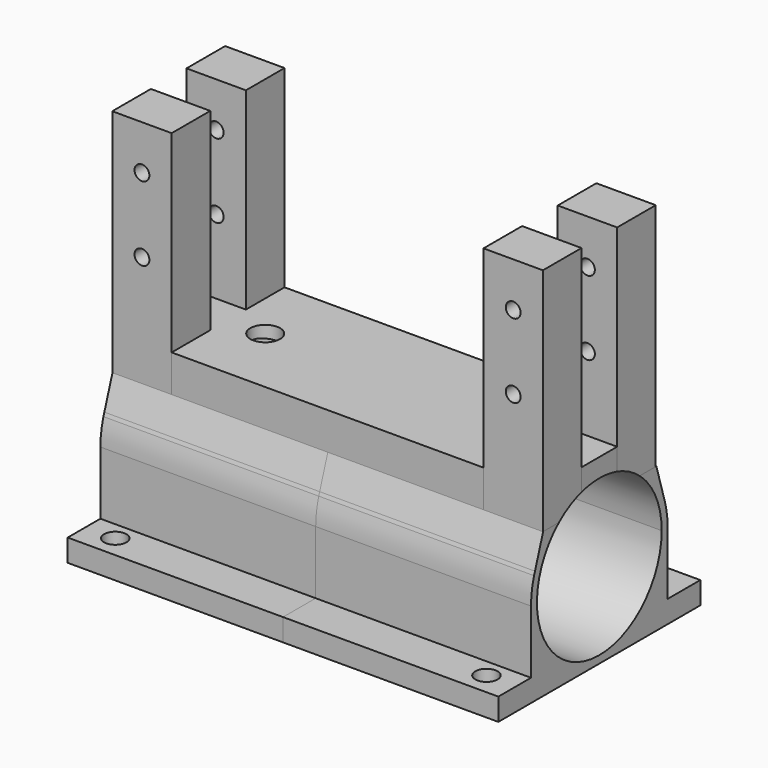
from build123d import *

# Parameters (mm, degrees)
F0_W      = 8
F0_H      = 6.5
F1_DEPTH  = 31
F0_R      = 2
F2_DEPTH  = 5
F3_R      = 1
F4_DEPTH  = 12.5
F5_W      = 5.5
F5_H      = 3
F6_DEPTH  = 29
F9_R      = 10.5
F10_DEPTH = 83.001
F0_R_2    = 1.5
F11_DEPTH = 19.501


# Not quite as in the source:
# - the program builds the solid bodies; features that only make, move or delete a surface that nothing else refers to are left out


with BuildPart() as f1:
    # F0 (on Top) → F1 (new body)
    with BuildSketch(Plane.XY):
        with Locations((-25, 6.25)):
            Rectangle(F0_W, F0_H)
    extrude(amount=F1_DEPTH)


with BuildPart() as f1b:
    # F0 (on Top) → F1, piece 2 (new body)
    with BuildSketch(Plane.XY):
        with Locations((-25, -6.25)):
            Rectangle(F0_W, F0_H)
    extrude(amount=F1_DEPTH)


with BuildPart() as f1c:
    # F0 (on Top) → F1, piece 3 (new body)
    with BuildSketch(Plane.XY):
        with Locations((25, 6.25)):
            Rectangle(F0_W, F0_H)
    extrude(amount=F1_DEPTH)


with BuildPart() as f1d:
    # F0 (on Top) → F1, piece 4 (new body)
    with BuildSketch(Plane.XY):
        with Locations((25, -6.25)):
            Rectangle(F0_W, F0_H)
    extrude(amount=F1_DEPTH)


with BuildPart() as f2:
    # F0 (on Top) → F2 (new body)
    with BuildSketch(Plane.XY):
        Polygon((-21, -9.5), (21, -9.5), (21, -3), (29, -3), (29, 3), (21, 3), (21, 9.5), (-21, 9.5), (-21, 3), (-29, 3), (-29, -3), (-21, -3), align=None)
        with Locations((-16, 0)):
            Circle(F0_R, mode=Mode.SUBTRACT)
        with Locations((16, 0)):
            Circle(F0_R, mode=Mode.SUBTRACT)
    extrude(amount=F2_DEPTH)


with BuildPart() as f4_tool:
    # F3 (on Front) → F4 (new body, symmetric)
    with BuildSketch(Plane.XZ):
        with Locations((25, 25)):
            Circle(F3_R)
        with Locations((25, 15)):
            Circle(F3_R)
        with Locations((-25, 25)):
            Circle(F3_R)
        with Locations((-25, 15)):
            Circle(F3_R)
    extrude(amount=F4_DEPTH, both=True)


with BuildPart() as f1_1:
    add(f1.part)

    # F4: cut by f4_tool
    add(f4_tool.part, mode=Mode.SUBTRACT)


with BuildPart() as f1b_1:
    add(f1b.part)

    # F4: cut by f4_tool
    add(f4_tool.part, mode=Mode.SUBTRACT)


with BuildPart() as f1c_1:
    add(f1c.part)

    # F4: cut by f4_tool
    add(f4_tool.part, mode=Mode.SUBTRACT)


with BuildPart() as f1d_1:
    add(f1d.part)

    # F4: cut by f4_tool
    add(f4_tool.part, mode=Mode.SUBTRACT)


with BuildPart() as f6:
    # F5 (on Right) → F6 (new body, symmetric)
    with BuildSketch(Plane.YZ):
        with BuildLine():
            ThreePointArc((-10.8310090403, -4.1348682857), (-9.7674911279, -1.9298997482), (-8.2613558209, 0))
            Line((-8.2613558209, 0), (-9.4548137859, 0))
            Line((-9.4548137859, 0), (-10.8310090403, -4.1348682857))
        make_face()
        with BuildLine():
            ThreePointArc((6.8007352544, 0), (9.5304176239, -3.5930577591), (10.5, -8))
            ThreePointArc((10.5, -8), (-4.4069422409, -17.5304176239), (-6.8007352544, 0))
            Line((-6.8007352544, 0), (-8.2613558209, 0))
            ThreePointArc((-8.2613558209, 0), (-9.7674911279, -1.9298997482), (-10.8310090403, -4.1348682857))
            Line((-10.8310090403, -4.1348682857), (-10.9869876699, -4.6035162385))
            ThreePointArc((-10.9869876699, -4.6035162385), (-11.3710236611, -6.2824957356), (-11.5, -8))
            ThreePointArc((-11.5, -8), (-8.1317279836, -16.1317279836), (0, -19.5))
            ThreePointArc((0, -19.5), (8.1317279836, -16.1317279836), (11.5, -8))
            ThreePointArc((11.5, -8), (11.3918398808, -6.4264739816), (11.0693940642, -4.8825467043))
            Line((11.0693940642, -4.8825467043), (10.9543418745, -4.499658003))
            ThreePointArc((10.9543418745, -4.499658003), (9.8677499977, -2.0942815862), (8.2613558209, 0))
            Line((8.2613558209, 0), (6.8007352544, 0))
        make_face()
        with BuildLine():
            Line((9.6022635698, 0), (8.2613558209, 0))
            ThreePointArc((8.2613558209, 0), (9.8677499977, -2.0942815862), (10.9543418745, -4.499658003))
            Line((10.9543418745, -4.499658003), (9.6022635698, 0))
        make_face()
        with BuildLine():
            ThreePointArc((6.8007352544, 0), (9.5304176239, -3.5930577591), (10.5, -8))
            ThreePointArc((10.5, -8), (-4.4069422409, -17.5304176239), (-6.8007352544, 0))
            Line((-6.8007352544, 0), (-8.2613558209, 0))
            ThreePointArc((-8.2613558209, 0), (-9.7674911279, -1.9298997482), (-10.8310090403, -4.1348682857))
            Line((-10.8310090403, -4.1348682857), (-10.9869876699, -4.6035162385))
            ThreePointArc((-10.9869876699, -4.6035162385), (-11.3710236611, -6.2824957356), (-11.5, -8))
            ThreePointArc((-11.5, -8), (-8.1317279836, -16.1317279836), (0, -19.5))
            ThreePointArc((0, -19.5), (8.1317279836, -16.1317279836), (11.5, -8))
            ThreePointArc((11.5, -8), (11.3918398808, -6.4264739816), (11.0693940642, -4.8825467043))
            Line((11.0693940642, -4.8825467043), (10.9543418745, -4.499658003))
            ThreePointArc((10.9543418745, -4.499658003), (9.8677499977, -2.0942815862), (8.2613558209, 0))
            Line((8.2613558209, 0), (6.8007352544, 0))
        make_face()
        with BuildLine():
            ThreePointArc((-6.8007352544, 0), (0, 2.5), (6.8007352544, 0))
            Line((6.8007352544, 0), (8.2613558209, 0))
            ThreePointArc((8.2613558209, 0), (0, 3.5), (-8.2613558209, 0))
            Line((-8.2613558209, 0), (-6.8007352544, 0))
        make_face()
        with BuildLine():
            ThreePointArc((6.8007352544, 0), (9.5304176239, -3.5930577591), (10.5, -8))
            ThreePointArc((10.5, -8), (-4.4069422409, -17.5304176239), (-6.8007352544, 0))
            Line((-6.8007352544, 0), (-8.2613558209, 0))
            ThreePointArc((-8.2613558209, 0), (-9.7674911279, -1.9298997482), (-10.8310090403, -4.1348682857))
            Line((-10.8310090403, -4.1348682857), (-10.9869876699, -4.6035162385))
            ThreePointArc((-10.9869876699, -4.6035162385), (-11.3710236611, -6.2824957356), (-11.5, -8))
            ThreePointArc((-11.5, -8), (-8.1317279836, -16.1317279836), (0, -19.5))
            ThreePointArc((0, -19.5), (8.1317279836, -16.1317279836), (11.5, -8))
            ThreePointArc((11.5, -8), (11.3918398808, -6.4264739816), (11.0693940642, -4.8825467043))
            Line((11.0693940642, -4.8825467043), (10.9543418745, -4.499658003))
            ThreePointArc((10.9543418745, -4.499658003), (9.8677499977, -2.0942815862), (8.2613558209, 0))
            Line((8.2613558209, 0), (6.8007352544, 0))
        make_face()
        with BuildLine():
            Line((11.5, -16.5), (11.5, -8))
            ThreePointArc((11.5, -8), (8.1317279836, -16.1317279836), (0, -19.5))
            Line((0, -19.5), (11.5, -19.5))
            Line((11.5, -19.5), (11.5, -16.5))
        make_face()
        with BuildLine():
            ThreePointArc((0, -19.5), (-8.1317279836, -16.1317279836), (-11.5, -8))
            Line((-11.5, -8), (-11.5, -16.5))
            Line((-11.5, -16.5), (-11.5, -19.5))
            Line((-11.5, -19.5), (0, -19.5))
        make_face()
        with Locations((-14.25, -18)):
            Rectangle(F5_W, F5_H)
        with Locations((14.25, -18)):
            Rectangle(F5_W, F5_H)
        with BuildLine():
            ThreePointArc((-6.8007352544, 0), (0, 2.5), (6.8007352544, 0))
            Line((6.8007352544, 0), (8.2613558209, 0))
            ThreePointArc((8.2613558209, 0), (0, 3.5), (-8.2613558209, 0))
            Line((-8.2613558209, 0), (-6.8007352544, 0))
        make_face()
    extrude(amount=F6_DEPTH, both=True)

    # F0 (on Top) → F11 (cut, through all)
    with BuildSketch(Plane.XY):
        with Locations((-25, -14)):
            Circle(F0_R_2)
        with Locations((25, -14)):
            Circle(F0_R_2)
        with Locations((-25, 14)):
            Circle(F0_R_2)
        with Locations((25, 14)):
            Circle(F0_R_2)
    extrude(amount=-F11_DEPTH, mode=Mode.SUBTRACT)


with BuildPart() as f10_tool:
    # F9 (on offset) → F10 (new body, through all)
    with BuildSketch(Plane.YZ.offset(54)):
        with Locations((0, -8)):
            Circle(F9_R)
    extrude(amount=-F10_DEPTH)


with BuildPart() as f1_2:
    add(f1_1.part)

    # F10: cut by f10_tool
    add(f10_tool.part, mode=Mode.SUBTRACT)


with BuildPart() as f1b_2:
    add(f1b_1.part)

    # F10: cut by f10_tool
    add(f10_tool.part, mode=Mode.SUBTRACT)


with BuildPart() as f1c_2:
    add(f1c_1.part)

    # F10: cut by f10_tool
    add(f10_tool.part, mode=Mode.SUBTRACT)


with BuildPart() as f1d_2:
    add(f1d_1.part)

    # F10: cut by f10_tool
    add(f10_tool.part, mode=Mode.SUBTRACT)


with BuildPart() as f2_1:
    add(f2.part)

    # F10: cut by f10_tool
    add(f10_tool.part, mode=Mode.SUBTRACT)


solid = Compound([f6.part, f1_2.part, f1b_2.part, f1c_2.part, f1d_2.part, f2_1.part])
